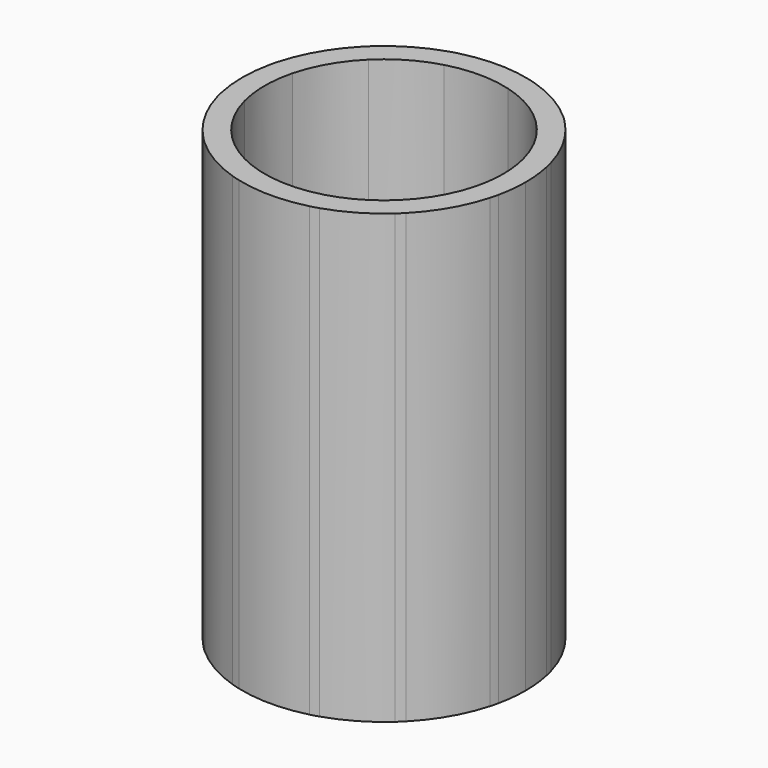
from build123d import *
from build123d import SkipClean  # not in build123d's __all__

# Parameters (mm, degrees)
F1_DEPTH = 30
F2_R     = 8
F3_DEPTH = 12


with BuildPart() as f1:
    # F0 (on Top) → F1 (new body)
    with BuildSketch(Plane.XY):
        with BuildLine():
            Line((-5.9997200782, 5.2918200067), (-6.7840477888, 6.6503154511))
            ThreePointArc((-6.7840477888, 6.6503154511), (-8.227241336, 4.75), (-9.1513660183, 2.55))
            Line((-9.1513660183, 2.55), (-7.5827105971, 2.55))
            ThreePointArc((-7.5827105971, 2.55), (-6.9282032303, 4), (-5.9997200782, 5.2918200067))
        make_face()
        with BuildLine():
            Line((-7.5827105971, 2.55), (-9.1513660183, 2.55))
            ThreePointArc((-9.1513660183, 2.55), (-9.2233274852, 2.2760118851), (-9.2870878105, 2))
            Line((-9.2870878105, 2), (-7.7459666924, 2))
            ThreePointArc((-7.7459666924, 2), (-7.6692706212, 2.2764639549), (-7.5827105971, 2.55))
        make_face()
        with BuildLine():
            Line((-7.7459666924, 2), (-9.2870878105, 2))
            ThreePointArc((-9.2870878105, 2), (-9.5, 0), (-9.2870878105, -2))
            Line((-9.2870878105, -2), (-7.7459666924, -2))
            ThreePointArc((-7.7459666924, -2), (-8, 0), (-7.7459666924, 2))
        make_face()
        with BuildLine():
            ThreePointArc((-9.2870878105, -2), (-9.2233274852, -2.2760118851), (-9.1513660183, -2.55))
            Line((-9.1513660183, -2.55), (-7.5827105971, -2.55))
            ThreePointArc((-7.5827105971, -2.55), (-7.6692706212, -2.2764639549), (-7.7459666924, -2))
            Line((-7.7459666924, -2), (-9.2870878105, -2))
        make_face()
        with BuildLine():
            ThreePointArc((-9.1513660183, -2.55), (-8.227241336, -4.75), (-6.7840477888, -6.6503154511))
            Line((-6.7840477888, -6.6503154511), (-5.9997200782, -5.2918200067))
            ThreePointArc((-5.9997200782, -5.2918200067), (-6.9282032303, -4), (-7.5827105971, -2.55))
            Line((-7.5827105971, -2.55), (-9.1513660183, -2.55))
        make_face()
        with BuildLine():
            ThreePointArc((-6.7840477888, -6.6503154511), (-6.5827478544, -6.849629967), (-6.3755947128, -7.0428539711))
            Line((-6.3755947128, -7.0428539711), (-5.6050341538, -5.7082039325))
            ThreePointArc((-5.6050341538, -5.7082039325), (-5.8061109264, -5.503551209), (-5.9997200782, -5.2918200067))
            Line((-5.9997200782, -5.2918200067), (-6.7840477888, -6.6503154511))
        make_face()
        with BuildLine():
            ThreePointArc((-6.3755947128, -7.0428539711), (-4.75, -8.227241336), (-2.9114930977, -9.0428539711))
            Line((-2.9114930977, -9.0428539711), (-2.1409325386, -7.7082039325))
            ThreePointArc((-2.1409325386, -7.7082039325), (-4, -6.9282032303), (-5.6050341538, -5.7082039325))
            Line((-5.6050341538, -5.7082039325), (-6.3755947128, -7.0428539711))
        make_face()
        with BuildLine():
            ThreePointArc((-2.9114930977, -9.0428539711), (-2.6405796308, -9.1256418521), (-2.3673182295, -9.2003154511))
            Line((-2.3673182295, -9.2003154511), (-1.5829905189, -7.8418200067))
            ThreePointArc((-1.5829905189, -7.8418200067), (-1.8631596948, -7.780015164), (-2.1409325386, -7.7082039325))
            Line((-2.1409325386, -7.7082039325), (-2.9114930977, -9.0428539711))
        make_face()
        with BuildLine():
            ThreePointArc((-2.3673182295, -9.2003154511), (0, -9.5), (2.3673182295, -9.2003154511))
            Line((2.3673182295, -9.2003154511), (1.5829905189, -7.8418200067))
            ThreePointArc((1.5829905189, -7.8418200067), (0, -8), (-1.5829905189, -7.8418200067))
            Line((-1.5829905189, -7.8418200067), (-2.3673182295, -9.2003154511))
        make_face()
        with BuildLine():
            ThreePointArc((2.3673182295, -9.2003154511), (2.6405796308, -9.1256418521), (2.9114930977, -9.0428539711))
            Line((2.9114930977, -9.0428539711), (2.1409325386, -7.7082039325))
            ThreePointArc((2.1409325386, -7.7082039325), (1.8631596948, -7.780015164), (1.5829905189, -7.8418200067))
            Line((1.5829905189, -7.8418200067), (2.3673182295, -9.2003154511))
        make_face()
        with BuildLine():
            ThreePointArc((2.9114930977, -9.0428539711), (4.75, -8.227241336), (6.3755947128, -7.0428539711))
            Line((6.3755947128, -7.0428539711), (5.6050341538, -5.7082039325))
            ThreePointArc((5.6050341538, -5.7082039325), (4, -6.9282032303), (2.1409325386, -7.7082039325))
            Line((2.1409325386, -7.7082039325), (2.9114930977, -9.0428539711))
        make_face()
        with BuildLine():
            ThreePointArc((6.3755947128, -7.0428539711), (6.5827478544, -6.849629967), (6.7840477888, -6.6503154511))
            Line((6.7840477888, -6.6503154511), (5.9997200782, -5.2918200067))
            ThreePointArc((5.9997200782, -5.2918200067), (5.8061109264, -5.503551209), (5.6050341538, -5.7082039325))
            Line((5.6050341538, -5.7082039325), (6.3755947128, -7.0428539711))
        make_face()
        with BuildLine():
            ThreePointArc((6.7840477888, -6.6503154511), (8.227241336, -4.75), (9.1513660183, -2.55))
            Line((9.1513660183, -2.55), (7.5827105971, -2.55))
            ThreePointArc((7.5827105971, -2.55), (6.9282032303, -4), (5.9997200782, -5.2918200067))
            Line((5.9997200782, -5.2918200067), (6.7840477888, -6.6503154511))
        make_face()
        with BuildLine():
            ThreePointArc((9.1513660183, -2.55), (9.2233274852, -2.2760118851), (9.2870878105, -2))
            Line((9.2870878105, -2), (7.7459666924, -2))
            ThreePointArc((7.7459666924, -2), (7.6692706212, -2.2764639549), (7.5827105971, -2.55))
            Line((7.5827105971, -2.55), (9.1513660183, -2.55))
        make_face()
        with BuildLine():
            ThreePointArc((9.2870878105, -2), (9.4466219941, -1.0056504861), (9.5, 0))
            ThreePointArc((9.5, 0), (9.4466219941, 1.0056504861), (9.2870878105, 2))
            Line((9.2870878105, 2), (7.7459666924, 2))
            ThreePointArc((7.7459666924, 2), (7.9362375701, 1.0080343399), (8, 0))
            ThreePointArc((8, 0), (7.9362375701, -1.0080343399), (7.7459666924, -2))
            Line((7.7459666924, -2), (9.2870878105, -2))
        make_face()
        with BuildLine():
            Line((7.7459666924, 2), (9.2870878105, 2))
            ThreePointArc((9.2870878105, 2), (9.2233274852, 2.2760118851), (9.1513660183, 2.55))
            Line((9.1513660183, 2.55), (7.5827105971, 2.55))
            ThreePointArc((7.5827105971, 2.55), (7.6692706212, 2.2764639549), (7.7459666924, 2))
        make_face()
        with BuildLine():
            Line((7.5827105971, 2.55), (9.1513660183, 2.55))
            ThreePointArc((9.1513660183, 2.55), (8.227241336, 4.75), (6.7840477888, 6.6503154511))
            Line((6.7840477888, 6.6503154511), (5.9997200782, 5.2918200067))
            ThreePointArc((5.9997200782, 5.2918200067), (6.9282032303, 4), (7.5827105971, 2.55))
        make_face()
        with BuildLine():
            Line((5.9997200782, 5.2918200067), (6.7840477888, 6.6503154511))
            ThreePointArc((6.7840477888, 6.6503154511), (6.5827478544, 6.849629967), (6.3755947128, 7.0428539711))
            Line((6.3755947128, 7.0428539711), (5.6050341538, 5.7082039325))
            ThreePointArc((5.6050341538, 5.7082039325), (5.8061109264, 5.503551209), (5.9997200782, 5.2918200067))
        make_face()
        with BuildLine():
            Line((5.6050341538, 5.7082039325), (6.3755947128, 7.0428539711))
            ThreePointArc((6.3755947128, 7.0428539711), (4.75, 8.227241336), (2.9114930977, 9.0428539711))
            Line((2.9114930977, 9.0428539711), (2.1409325386, 7.7082039325))
            ThreePointArc((2.1409325386, 7.7082039325), (4, 6.9282032303), (5.6050341538, 5.7082039325))
        make_face()
        with BuildLine():
            Line((2.1409325386, 7.7082039325), (2.9114930977, 9.0428539711))
            ThreePointArc((2.9114930977, 9.0428539711), (2.6405796308, 9.1256418521), (2.3673182295, 9.2003154511))
            Line((2.3673182295, 9.2003154511), (1.5829905189, 7.8418200067))
            ThreePointArc((1.5829905189, 7.8418200067), (1.8631596948, 7.780015164), (2.1409325386, 7.7082039325))
        make_face()
        with BuildLine():
            Line((1.5829905189, 7.8418200067), (2.3673182295, 9.2003154511))
            ThreePointArc((2.3673182295, 9.2003154511), (0, 9.5), (-2.3673182295, 9.2003154511))
            Line((-2.3673182295, 9.2003154511), (-1.5829905189, 7.8418200067))
            ThreePointArc((-1.5829905189, 7.8418200067), (0, 8), (1.5829905189, 7.8418200067))
        make_face()
        with BuildLine():
            Line((-1.5829905189, 7.8418200067), (-2.3673182295, 9.2003154511))
            ThreePointArc((-2.3673182295, 9.2003154511), (-2.6405796308, 9.1256418521), (-2.9114930977, 9.0428539711))
            Line((-2.9114930977, 9.0428539711), (-2.1409325386, 7.7082039325))
            ThreePointArc((-2.1409325386, 7.7082039325), (-1.8631596948, 7.780015164), (-1.5829905189, 7.8418200067))
        make_face()
        with BuildLine():
            Line((-2.1409325386, 7.7082039325), (-2.9114930977, 9.0428539711))
            ThreePointArc((-2.9114930977, 9.0428539711), (-4.75, 8.227241336), (-6.3755947128, 7.0428539711))
            Line((-6.3755947128, 7.0428539711), (-5.6050341538, 5.7082039325))
            ThreePointArc((-5.6050341538, 5.7082039325), (-4, 6.9282032303), (-2.1409325386, 7.7082039325))
        make_face()
        with BuildLine():
            Line((-5.6050341538, 5.7082039325), (-6.3755947128, 7.0428539711))
            ThreePointArc((-6.3755947128, 7.0428539711), (-6.5827478544, 6.849629967), (-6.7840477888, 6.6503154511))
            Line((-6.7840477888, 6.6503154511), (-5.9997200782, 5.2918200067))
            ThreePointArc((-5.9997200782, 5.2918200067), (-5.8061109264, 5.503551209), (-5.6050341538, 5.7082039325))
        make_face()
        with BuildLine():
            Line((1.4722431864, 7.65), (1.5829905189, 7.8418200067))
            ThreePointArc((1.5829905189, 7.8418200067), (0, 8), (-1.5829905189, 7.8418200067))
            Line((-1.5829905189, 7.8418200067), (-1.4722431864, 7.65))
            Line((-1.4722431864, 7.65), (1.4722431864, 7.65))
        make_face()
        with BuildLine():
            Line((-7.3612159322, 2.55), (-5.8889727457, 5.1))
            Line((-5.8889727457, 5.1), (-5.9997200782, 5.2918200067))
            ThreePointArc((-5.9997200782, 5.2918200067), (-6.9282032303, 4), (-7.5827105971, 2.55))
            Line((-7.5827105971, 2.55), (-7.3612159322, 2.55))
        make_face()
        with BuildLine():
            Line((-5.9997200782, -5.2918200067), (-5.8889727457, -5.1))
            Line((-5.8889727457, -5.1), (-7.3612159322, -2.55))
            Line((-7.3612159322, -2.55), (-7.5827105971, -2.55))
            ThreePointArc((-7.5827105971, -2.55), (-6.9282032303, -4), (-5.9997200782, -5.2918200067))
        make_face()
        with BuildLine():
            ThreePointArc((-1.5829905189, -7.8418200067), (0, -8), (1.5829905189, -7.8418200067))
            Line((1.5829905189, -7.8418200067), (1.4722431864, -7.65))
            Line((1.4722431864, -7.65), (-1.4722431864, -7.65))
            Line((-1.4722431864, -7.65), (-1.5829905189, -7.8418200067))
        make_face()
        with BuildLine():
            ThreePointArc((5.9997200782, -5.2918200067), (6.9282032303, -4), (7.5827105971, -2.55))
            Line((7.5827105971, -2.55), (7.3612159322, -2.55))
            Line((7.3612159322, -2.55), (5.8889727457, -5.1))
            Line((5.8889727457, -5.1), (5.9997200782, -5.2918200067))
        make_face()
        with BuildLine():
            Line((7.3612159322, 2.55), (7.5827105971, 2.55))
            ThreePointArc((7.5827105971, 2.55), (6.9282032303, 4), (5.9997200782, 5.2918200067))
            Line((5.9997200782, 5.2918200067), (5.8889727457, 5.1))
            Line((5.8889727457, 5.1), (7.3612159322, 2.55))
        make_face()
        with BuildLine():
            Line((5.8889727457, 5.1), (5.9997200782, 5.2918200067))
            ThreePointArc((5.9997200782, 5.2918200067), (5.8061109264, 5.503551209), (5.6050341538, 5.7082039325))
            Line((5.6050341538, 5.7082039325), (5.5714300977, 5.65))
            Line((5.5714300977, 5.65), (3.2620290209, 5.65))
            Line((3.2620290209, 5.65), (2.1073284825, 7.65))
            Line((2.1073284825, 7.65), (2.1409325386, 7.7082039325))
            ThreePointArc((2.1409325386, 7.7082039325), (1.8631596948, 7.780015164), (1.5829905189, 7.8418200067))
            Line((1.5829905189, 7.8418200067), (1.4722431864, 7.65))
            Line((1.4722431864, 7.65), (2.9444863729, 5.1))
            Line((2.9444863729, 5.1), (5.8889727457, 5.1))
        make_face()
        with BuildLine():
            Line((-1.4722431864, 7.65), (-1.5829905189, 7.8418200067))
            ThreePointArc((-1.5829905189, 7.8418200067), (-1.8631596948, 7.780015164), (-2.1409325386, 7.7082039325))
            Line((-2.1409325386, 7.7082039325), (-2.1073284825, 7.65))
            Line((-2.1073284825, 7.65), (-3.2620290209, 5.65))
            Line((-3.2620290209, 5.65), (-5.5714300977, 5.65))
            Line((-5.5714300977, 5.65), (-5.6050341538, 5.7082039325))
            ThreePointArc((-5.6050341538, 5.7082039325), (-5.8061109264, 5.503551209), (-5.9997200782, 5.2918200067))
            Line((-5.9997200782, 5.2918200067), (-5.8889727457, 5.1))
            Line((-5.8889727457, 5.1), (-2.9444863729, 5.1))
            Line((-2.9444863729, 5.1), (-1.4722431864, 7.65))
        make_face()
        with BuildLine():
            Line((-7.3612159322, -2.55), (-5.8889727457, 0))
            Line((-5.8889727457, 0), (-7.3612159322, 2.55))
            Line((-7.3612159322, 2.55), (-7.5827105971, 2.55))
            ThreePointArc((-7.5827105971, 2.55), (-7.6692706212, 2.2764639549), (-7.7459666924, 2))
            Line((-7.7459666924, 2), (-7.6787585802, 2))
            Line((-7.6787585802, 2), (-6.5240580418, 0))
            Line((-6.5240580418, 0), (-7.6787585802, -2))
            Line((-7.6787585802, -2), (-7.7459666924, -2))
            ThreePointArc((-7.7459666924, -2), (-7.6692706212, -2.2764639549), (-7.5827105971, -2.55))
            Line((-7.5827105971, -2.55), (-7.3612159322, -2.55))
        make_face()
        with BuildLine():
            Line((7.6787585802, 2), (7.7459666924, 2))
            ThreePointArc((7.7459666924, 2), (7.6692706212, 2.2764639549), (7.5827105971, 2.55))
            Line((7.5827105971, 2.55), (7.3612159322, 2.55))
            Line((7.3612159322, 2.55), (5.8889727457, 0))
            Line((5.8889727457, 0), (7.3612159322, -2.55))
            Line((7.3612159322, -2.55), (7.5827105971, -2.55))
            ThreePointArc((7.5827105971, -2.55), (7.6692706212, -2.2764639549), (7.7459666924, -2))
            Line((7.7459666924, -2), (7.6787585802, -2))
            Line((7.6787585802, -2), (6.5240580418, 0))
            Line((6.5240580418, 0), (7.6787585802, 2))
        make_face()
        with BuildLine():
            ThreePointArc((5.6050341538, -5.7082039325), (5.8061109264, -5.503551209), (5.9997200782, -5.2918200067))
            Line((5.9997200782, -5.2918200067), (5.8889727457, -5.1))
            Line((5.8889727457, -5.1), (2.9444863729, -5.1))
            Line((2.9444863729, -5.1), (1.4722431864, -7.65))
            Line((1.4722431864, -7.65), (1.5829905189, -7.8418200067))
            ThreePointArc((1.5829905189, -7.8418200067), (1.8631596948, -7.780015164), (2.1409325386, -7.7082039325))
            Line((2.1409325386, -7.7082039325), (2.1073284825, -7.65))
            Line((2.1073284825, -7.65), (3.2620290209, -5.65))
            Line((3.2620290209, -5.65), (5.5714300977, -5.65))
            Line((5.5714300977, -5.65), (5.6050341538, -5.7082039325))
        make_face()
        with BuildLine():
            ThreePointArc((-2.1409325386, -7.7082039325), (-1.8631596948, -7.780015164), (-1.5829905189, -7.8418200067))
            Line((-1.5829905189, -7.8418200067), (-1.4722431864, -7.65))
            Line((-1.4722431864, -7.65), (-2.9444863729, -5.1))
            Line((-2.9444863729, -5.1), (-5.8889727457, -5.1))
            Line((-5.8889727457, -5.1), (-5.9997200782, -5.2918200067))
            ThreePointArc((-5.9997200782, -5.2918200067), (-5.8061109264, -5.503551209), (-5.6050341538, -5.7082039325))
            Line((-5.6050341538, -5.7082039325), (-5.5714300977, -5.65))
            Line((-5.5714300977, -5.65), (-3.2620290209, -5.65))
            Line((-3.2620290209, -5.65), (-2.1073284825, -7.65))
            Line((-2.1073284825, -7.65), (-2.1409325386, -7.7082039325))
        make_face()
        Polygon((-2.9444863729, -5.1), (-1.4722431864, -2.55), (-2.9444863729, 0), (-5.8889727457, 0), (-7.3612159322, -2.55), (-5.8889727457, -5.1), align=None)
        Polygon((-5.5714300977, -0.55), (-3.2620290209, -0.55), (-2.1073284825, -2.55), (-3.2620290209, -4.55), (-5.5714300977, -4.55), (-6.7261306361, -2.55), align=None, mode=Mode.SUBTRACT)
        Polygon((1.4722431864, -7.65), (2.9444863729, -5.1), (1.4722431864, -2.55), (-1.4722431864, -2.55), (-2.9444863729, -5.1), (-1.4722431864, -7.65), align=None)
        Polygon((1.1547005384, -7.1), (-1.1547005384, -7.1), (-2.3094010768, -5.1), (-1.1547005384, -3.1), (1.1547005384, -3.1), (2.3094010768, -5.1), align=None, mode=Mode.SUBTRACT)
        Polygon((5.8889727457, -5.1), (7.3612159322, -2.55), (5.8889727457, 0), (2.9444863729, 0), (1.4722431864, -2.55), (2.9444863729, -5.1), align=None)
        Polygon((5.5714300977, -4.55), (3.2620290209, -4.55), (2.1073284825, -2.55), (3.2620290209, -0.55), (5.5714300977, -0.55), (6.7261306361, -2.55), align=None, mode=Mode.SUBTRACT)
        Polygon((5.8889727457, 0), (7.3612159322, 2.55), (5.8889727457, 5.1), (2.9444863729, 5.1), (1.4722431864, 2.55), (2.9444863729, 0), align=None)
        Polygon((5.5714300977, 4.55), (6.7261306361, 2.55), (5.5714300977, 0.55), (3.2620290209, 0.55), (2.1073284825, 2.55), (3.2620290209, 4.55), align=None, mode=Mode.SUBTRACT)
        Polygon((1.4722431864, 2.55), (2.9444863729, 5.1), (1.4722431864, 7.65), (-1.4722431864, 7.65), (-2.9444863729, 5.1), (-1.4722431864, 2.55), align=None)
        Polygon((1.1547005384, 7.1), (2.3094010768, 5.1), (1.1547005384, 3.1), (-1.1547005384, 3.1), (-2.3094010768, 5.1), (-1.1547005384, 7.1), align=None, mode=Mode.SUBTRACT)
        Polygon((-2.9444863729, 0), (-1.4722431864, 2.55), (-2.9444863729, 5.1), (-5.8889727457, 5.1), (-7.3612159322, 2.55), (-5.8889727457, 0), align=None)
        Polygon((-3.2620290209, 4.55), (-2.1073284825, 2.55), (-3.2620290209, 0.55), (-5.5714300977, 0.55), (-6.7261306361, 2.55), (-5.5714300977, 4.55), align=None, mode=Mode.SUBTRACT)
        Polygon((1.4722431864, -2.55), (2.9444863729, 0), (1.4722431864, 2.55), (-1.4722431864, 2.55), (-2.9444863729, 0), (-1.4722431864, -2.55), align=None)
        Polygon((1.1547005384, 2), (2.3094010768, 0), (1.1547005384, -2), (-1.1547005384, -2), (-2.3094010768, 0), (-1.1547005384, 2), align=None, mode=Mode.SUBTRACT)
    extrude(amount=-F1_DEPTH)

    # F2 (on Top) → F3 (cut)
    with BuildSketch(Plane.XY):
        Circle(F2_R)
    with SkipClean():  # cleaning this boolean's faces spoils the solid; the shape is the same uncleaned
        extrude(amount=-F3_DEPTH, mode=Mode.SUBTRACT)


solid = f1.part
